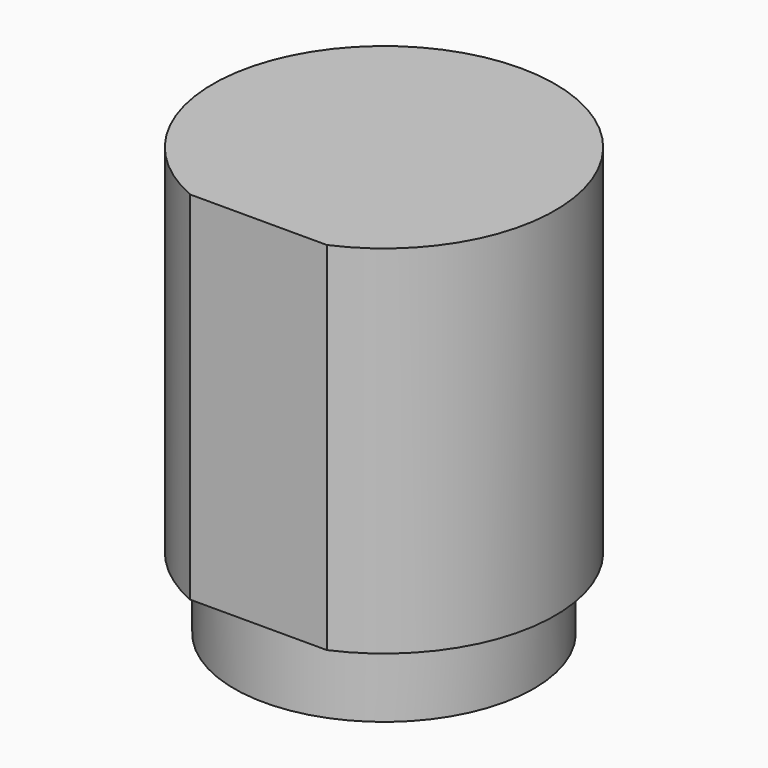
from build123d import *

# Parameters (mm, degrees)
F3_DEPTH = 25


# Not quite as in the source:
# - a feature names something its author has since deleted; it is built from what else it names


with BuildPart() as f1:
    # F0 (on Front) → F1 (revolve)
    with BuildSketch(Plane.XZ):
        with BuildLine():
            Line((-12, -25), (-10.5, -25))
            Line((-10.5, -25), (-10.5, -30))
            Line((-10.5, -30), (-9, -30))
            Line((-9, -30), (-9, -7.2415010072))
            ThreePointArc((-9, -7.2415010072), (-4.9914312836, -4.0779872119), (0, -3))
            Line((0, -3), (0, 0))
            Line((0, 0), (-3, 0))
            Line((-3, 0), (-12, 0))
            Line((-12, 0), (-12, -3))
            Line((-12, -3), (-12, -25))
        make_face()
    revolve(axis=Axis((0, 0, -1.5), (0, 0, -1)))

    # F2 (on face) → F3 (cut)
    with BuildSketch(Plane(origin=(0, 0, -25), x_dir=(1, 0, 0), z_dir=(0, 0, -1))):
        Polygon((-5, 11), (0, 11), (5, 11), (5, 12.7678344972), (0, 12.7678344972), (-5, 12.7678344972), align=None)
    extrude(amount=-F3_DEPTH, mode=Mode.SUBTRACT)


solid = f1.part
